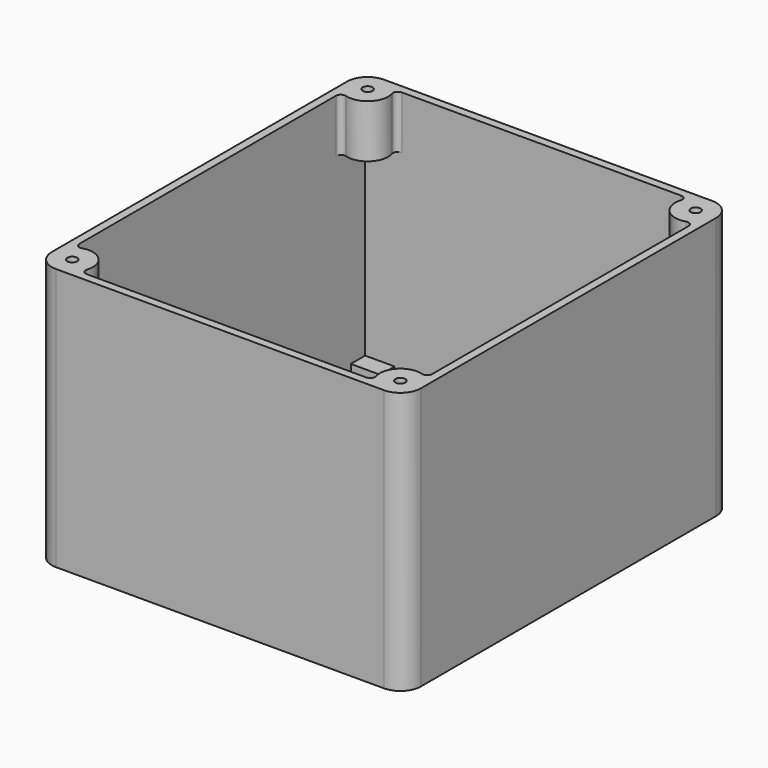
from build123d import *

# Parameters (mm, degrees)
F0_R     = 1.524
F1_DEPTH = 81.28
F2_W     = 13.3946808136
F2_H     = 17.3983402467
F2_W_2   = 15.2697945094
F2_H_2   = 13.5166846132
F3_DEPTH = 64.8716
F5_DEPTH = 5.842


# Not quite as in the source:
# - ends of sketch curves that miss each other by under 0.0002 mm in the source are joined


with BuildPart() as f1:
    # F0 (on Top) → F1 (new body)
    with BuildSketch(Plane.XY):
        with BuildLine():
            Line((57.15, -57.15), (57.15, 57.15))
            ThreePointArc((57.15, 57.15), (55.2901280605, 61.6401280605), (50.8, 63.5))
            Line((50.8, 63.5), (-50.8, 63.5))
            ThreePointArc((-50.8, 63.5), (-55.2901280605, 61.6401280605), (-57.15, 57.15))
            Line((-57.15, 57.15), (-57.15, -57.15))
            ThreePointArc((-57.15, -57.15), (-55.2901280605, -61.6401280605), (-50.8, -63.5))
            Line((-50.8, -63.5), (50.8, -63.5))
            ThreePointArc((50.8, -63.5), (55.2901280605, -61.6401280605), (57.15, -57.15))
        make_face()
        with Locations((-50.8, -57.15)):
            Circle(F0_R, mode=Mode.SUBTRACT)
        with Locations((50.8, -57.15)):
            Circle(F0_R, mode=Mode.SUBTRACT)
        with Locations((-50.8, 57.15)):
            Circle(F0_R, mode=Mode.SUBTRACT)
        with BuildLine():
            Line((-43.2651408, 60.96), (43.2651408, 60.96))
            ThreePointArc((43.2651408, 60.96), (44.4892438959, 60.34382576), (44.7235034291, 58.993558544))
            ThreePointArc((44.7235034291, 58.993558544), (46.3098719395, 52.6598719395), (52.643558117, 51.0735048367))
            ThreePointArc((52.643558117, 51.0735048367), (53.99382576, 50.8392438959), (54.61, 49.6151408))
            Line((54.61, 49.6151408), (54.61, -49.6151408))
            ThreePointArc((54.61, -49.6151408), (53.99382576, -50.8392438959), (52.643558544, -51.0735034291))
            ThreePointArc((52.643558544, -51.0735034291), (46.3098719395, -52.6598719395), (44.7235048367, -58.993558117))
            ThreePointArc((44.7235048367, -58.993558117), (44.4892438959, -60.34382576), (43.2651408, -60.96))
            Line((43.2651408, -60.96), (-43.2651408, -60.96))
            ThreePointArc((-43.2651408, -60.96), (-44.4892438959, -60.34382576), (-44.7235034291, -58.993558544))
            ThreePointArc((-44.7235034291, -58.993558544), (-46.3098719395, -52.6598719395), (-52.643558117, -51.0735048367))
            ThreePointArc((-52.643558117, -51.0735048367), (-53.99382576, -50.8392438959), (-54.61, -49.6151408))
            Line((-54.61, -49.6151408), (-54.61, 49.6151408))
            ThreePointArc((-54.61, 49.6151408), (-53.99382576, 50.8392438959), (-52.643558544, 51.0735034291))
            ThreePointArc((-52.643558544, 51.0735034291), (-46.3098719395, 52.6598719395), (-44.7235048367, 58.993558117))
            ThreePointArc((-44.7235048367, 58.993558117), (-44.4892438959, 60.34382576), (-43.2651408, 60.96))
        make_face(mode=Mode.SUBTRACT)
        with Locations((50.8, 57.15)):
            Circle(F0_R, mode=Mode.SUBTRACT)
    extrude(amount=F1_DEPTH)

    # F2 (on face) → F3 (cut)
    with BuildSketch(Plane(origin=(0, 0, 0), x_dir=(1, 0, 0), z_dir=(0, 0, -1))):
        with Locations((47.9126595932, 52.2608298767)):
            Rectangle(F2_W, F2_H)
        Polygon((-54.61, 60.96), (-54.61, 45.5632209778), (-42.4256250262, 45.9913872182), (-42.4256250262, 60.96), align=None)
        Polygon((37.4062317246, -45.9566726098), (37.9334576428, -60.96), (54.61, -60.96), (54.61, -45.9566726098), align=None)
        with Locations((-46.9751027453, -54.2016576934)):
            Rectangle(F2_W_2, F2_H_2)
    extrude(amount=-F3_DEPTH, mode=Mode.SUBTRACT)

    # F4 (on Top) → F5 (join)
    with BuildSketch(Plane.XY):
        Polygon((-45.8822585642, -55.3943701088), (-55.0047931408, -55.3943701088), (-54.9012337958, -60.975112021), (-45.8822585642, -60.975112021), align=None)
        Polygon((-45.4961853886, 60.9891191125), (-54.7619216034, 60.9891191125), (-54.6583622584, 55.4083772004), (-45.4961853886, 55.4083772004), align=None)
        Polygon((54.7389825022, 60.9891191125), (45.6164479256, 60.9891191125), (45.7200072706, 55.4083772004), (54.7389825022, 55.4083772004), align=None)
        Polygon((54.6354231571, -55.3943701088), (45.5128885806, -55.3943701088), (45.6164479256, -60.975112021), (54.6354231571, -60.975112021), align=None)
    extrude(amount=F5_DEPTH)


solid = f1.part
